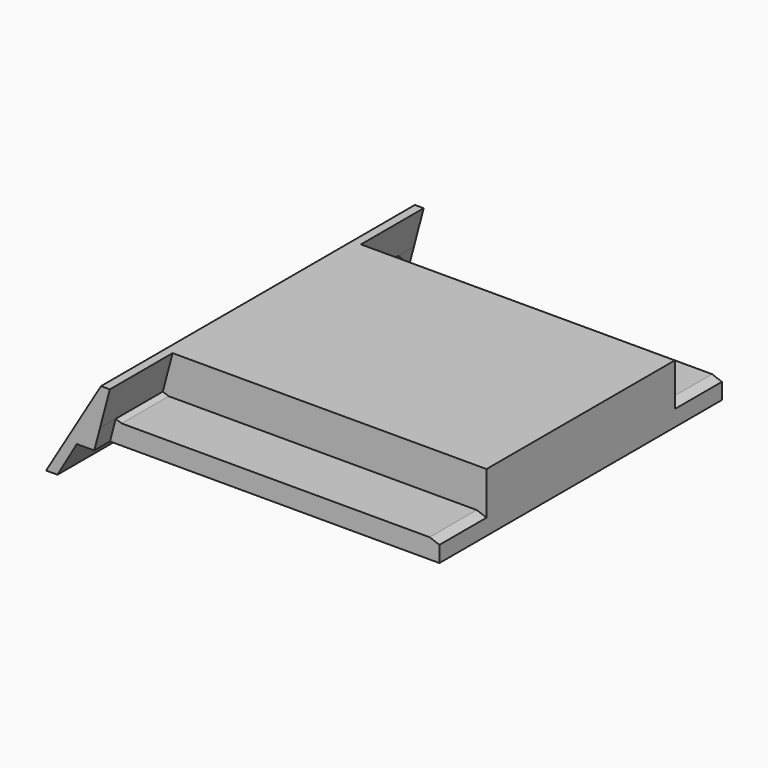
from build123d import *

# Parameters (mm, degrees)
F1_DEPTH  = 20
F3_DEPTH  = 4
F5_DEPTH  = 1
F7_DEPTH  = 20.001
F10_W     = 15
F10_H     = 9.1
F11_DEPTH = 1


# Not quite as in the source:
# - a pattern or mirror of a feature is missing from the dataset's text; its kind, count and spacing are read off the source's solid


with BuildPart() as f1:
    # F0 (on Front) → F1 (new body)
    with BuildSketch(Plane.XZ):
        Polygon((-16.45, 3), (-19.25, -1.7), (-18.09, -1.7), (-17.0772340426, 0), (0, 0), (0, 3), align=None)
    extrude(amount=F1_DEPTH)

    # F2 (on face) → F3 (cut)
    with BuildSketch(Plane.XZ.offset(20)):
        Polygon((-16.2, 1), (-0.5, 1), (0, 0.8180148829), (0, 3), (-16, 3), (-16.5, 1.1091910703), align=None)
    f3 = extrude(amount=-F3_DEPTH, mode=Mode.SUBTRACT)

    # F3_copies: F3 across plane
    add(f3.mirror(Plane.ZX.offset(-10)), mode=Mode.SUBTRACT)

    # F4 (on face) → F5 (cut)
    with BuildSketch(Plane.XZ.offset(20)):
        Polygon((0, -1), (0, 0.8180148829), (-0.5, 1), (-16.2, 1), (-16.5, 1.1091910703), (-17.0577483365, -1), align=None)
    f5 = extrude(amount=-F5_DEPTH, mode=Mode.SUBTRACT)

    # F5_copies: F5 across plane
    add(f5.mirror(Plane.ZX.offset(-10)), mode=Mode.SUBTRACT)

    # F6 (on face) → F7 (cut, through all)
    with BuildSketch(Plane.XZ.offset(20)):
        Polygon((-18.67, -1.7), (-18.09, -1.7), (-17.0772340426, 0), (-17.683862779, 0), align=None)
    extrude(amount=-F7_DEPTH, mode=Mode.SUBTRACT)

    # F10 (on face) → F11 (cut)
    with BuildSketch(Plane(origin=(0, 0, 0), x_dir=(1, 0, 0), z_dir=(0, 0, -1))):
        with Locations((-9, 10)):
            Rectangle(F10_W, F10_H)
    extrude(amount=-F11_DEPTH, mode=Mode.SUBTRACT)


solid = f1.part
